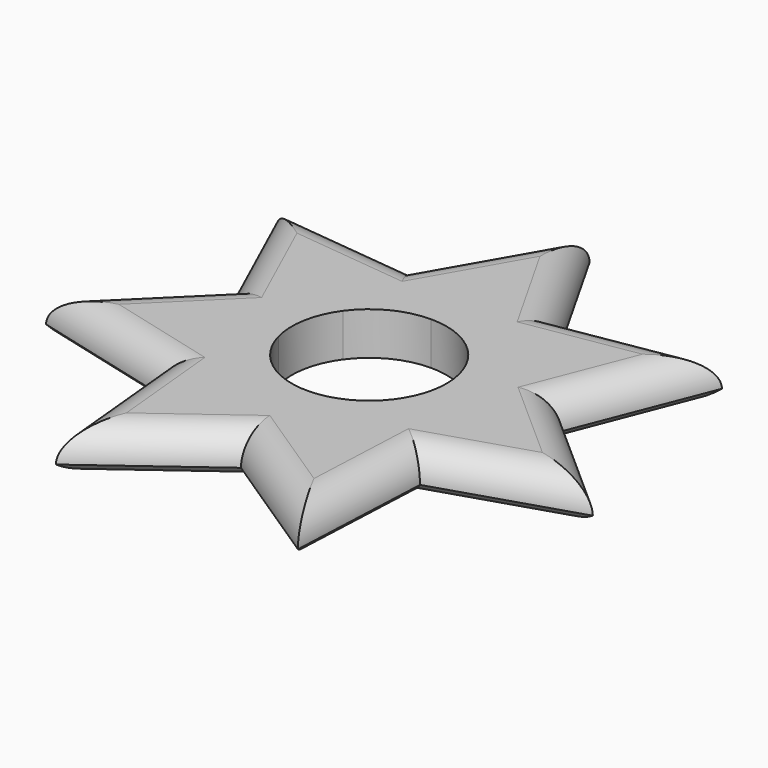
from build123d import *

# Parameters (mm, degrees)
F1_DEPTH      = 7
F2_R          = 5
F3_T4_DEPTH   = 43.6349666374
F3_T9_DEPTH   = 43.6349666374
F3_T14_DEPTH  = 44.4129734555
F3_T19_DEPTH  = 44.4129734555
F3_T24_DEPTH  = 43.6349666396
F3_T29_DEPTH  = 43.6349666396
F3_T34_DEPTH  = 43.6349666396
F3_T39_DEPTH  = 43.6349666396
F3_T44_DEPTH  = 43.6349666396
F3_T49_DEPTH  = 43.6349666396
F3_T54_DEPTH  = 43.6349666396
F3_T59_DEPTH  = 43.6349666418
F3_T64_DEPTH  = 43.6349666418
F3_T69_DEPTH  = 43.6349666396
F3_T75_DEPTH  = 43.6349666374
F3_T79_DEPTH  = 43.6349666374
F3_T86_DEPTH  = 44.4129734555
F3_T90_DEPTH  = 44.4129734555
F3_T97_DEPTH  = 43.6349666396
F3_T101_DEPTH = 43.6349666396
F3_T108_DEPTH = 43.6349666396
F3_T112_DEPTH = 43.6349666396
F3_T119_DEPTH = 43.6349666396
F3_T123_DEPTH = 43.6349666396
F3_T130_DEPTH = 43.6349666396
F3_T134_DEPTH = 43.6349666396
F3_T141_DEPTH = 43.6349666418
F3_T145_DEPTH = 43.6349666418


# Not quite as in the source:
# - a fillet or chamfer that OpenCascade refuses, or shapes differently, is made with other operations: its cross-section is extruded or revolved along the edge and cut away or added


with BuildPart() as f1:
    # F0 (on Top) → F1 (new body)
    with BuildSketch(Plane.XY):
        Polygon((20.4295724883, -40.0952935885), (10.2147862441, -20.0476467942), (0.70880785, -27.0682797275), align=None)
        Polygon((-18.3031489384, -41.1095455939), (-9.1515744692, -20.554772797), (-20.5899370405, -17.5854675412), align=None)
        Polygon((-20.5899370405, -17.5854675412), (-21.7333310915, -5.8234285148), (-43.466662183, -11.6468570296), align=None)
        Polygon((-12.1352549156, 23.8167787844), (0, 22.5), (0, 45), align=None)
        Polygon((-43.466662183, -11.6468570296), (-21.7333310915, -5.8234285148), (-26.62414231, 4.9344931078), align=None)
        Polygon((21.4820715071, -16.4837732251), (10.2147862441, -20.0476467942), (20.4295724883, -40.0952935885), align=None)
        Polygon((-26.62414231, 4.9344931078), (-18.2028823734, 13.2251681766), (-36.4057647469, 26.4503363532), align=None)
        with BuildLine():
            Line((10.2147862441, -20.0476467942), (7.7328428868, -15.176558687))
            ThreePointArc((7.7328428868, -15.176558687), (0.4458732697, -17.0272132106), (-6.927965583, -15.5604654677))
            Line((-6.927965583, -15.5604654677), (-9.1515744692, -20.554772797))
            Line((-9.1515744692, -20.554772797), (10.2147862441, -20.0476467942))
        make_face()
        Polygon((0, 45), (0, 22.5), (11.6571894205, 24.4398058675), align=None)
        Polygon((0.70880785, -27.0682797275), (-9.1515744692, -20.554772797), (-18.3031489384, -41.1095455939), align=None)
        Polygon((-18.2028823734, 13.2251681766), (0, 22.5), (-12.1352549156, 23.8167787844), align=None)
        with BuildLine():
            Line((7.7328428868, -15.176558687), (5.7403470363, -11.2660653986))
            ThreePointArc((5.7403470363, -11.2660653986), (0.3309865905, -12.63986794), (-5.1428597844, -11.5510521989))
            Line((-5.1428597844, -11.5510521989), (-6.927965583, -15.5604654677))
            ThreePointArc((-6.927965583, -15.5604654677), (0.4458732697, -17.0272132106), (7.7328428868, -15.176558687))
        make_face()
        Polygon((34.9715682614, 28.3194176024), (17.4857841307, 14.1597088012), (26.3294034315, 6.3211305052), align=None)
        Polygon((11.6571894205, 24.4398058675), (17.4857841307, 14.1597088012), (34.9715682614, 28.3194176024), align=None)
        Polygon((0, 22.5), (17.4857841307, 14.1597088012), (11.6571894205, 24.4398058675), align=None)
        with BuildLine():
            Line((16.6608370018, -3.5413702277), (12.3678946677, -2.6288771657))
            ThreePointArc((12.3678946677, -2.6288771657), (10.0313189335, -7.6973017427), (5.7403470363, -11.2660653986))
            Line((5.7403470363, -11.2660653986), (7.7328428868, -15.176558687))
            ThreePointArc((7.7328428868, -15.176558687), (13.5132271219, -10.3690638653), (16.6608370018, -3.5413702277))
        make_face()
        Polygon((44.016642033, -9.3560260868), (22.0083210165, -4.6780130434), (21.4820715071, -16.4837732251), align=None)
        Polygon((-20.5899370405, -17.5854675412), (-9.1515744692, -20.554772797), (-21.7333310915, -5.8234285148), align=None)
        Polygon((26.3294034315, 6.3211305052), (22.0083210165, -4.6780130434), (44.016642033, -9.3560260868), align=None)
        with BuildLine():
            ThreePointArc((-12.2133600976, -3.272559975), (-12.4324724808, 2.3042225757), (-10.2293733208, 7.4320747524))
            Line((-10.2293733208, 7.4320747524), (-13.7800269253, 10.0117755983))
            ThreePointArc((-13.7800269253, 10.0117755983), (-16.7478300145, 3.1040268196), (-16.4526629065, -4.4084777391))
            Line((-16.4526629065, -4.4084777391), (-12.2133600976, -3.272559975))
        make_face()
        with BuildLine():
            ThreePointArc((-16.4526629065, -4.4084777391), (-16.7478300145, 3.1040268196), (-13.7800269253, 10.0117755983))
            Line((-13.7800269253, 10.0117755983), (-18.2028823734, 13.2251681766))
            Line((-18.2028823734, 13.2251681766), (-21.7333310915, -5.8234285148))
            Line((-21.7333310915, -5.8234285148), (-16.4526629065, -4.4084777391))
        make_face()
        Polygon((0.70880785, -27.0682797275), (10.2147862441, -20.0476467942), (-9.1515744692, -20.554772797), align=None)
        with BuildLine():
            ThreePointArc((0, 12.6442007918), (5.4434687503, 11.4124695674), (9.82638958, 7.9572533883))
            Line((9.82638958, 7.9572533883), (13.2371660261, 10.7192456959))
            ThreePointArc((13.2371660261, 10.7192456959), (7.3329170413, 15.3737802884), (0, 17.0330500114))
            Line((0, 17.0330500114), (0, 12.6442007918))
        make_face()
        Polygon((-36.4057647469, 26.4503363532), (-18.2028823734, 13.2251681766), (-12.1352549156, 23.8167787844), align=None)
        with BuildLine():
            Line((22.0083210165, -4.6780130434), (16.6608370018, -3.5413702277))
            ThreePointArc((16.6608370018, -3.5413702277), (13.5132271219, -10.3690638653), (7.7328428868, -15.176558687))
            Line((7.7328428868, -15.176558687), (10.2147862441, -20.0476467942))
            Line((10.2147862441, -20.0476467942), (22.0083210165, -4.6780130434))
        make_face()
        with BuildLine():
            ThreePointArc((-10.2293733208, 7.4320747524), (-5.7403470363, 11.2660653986), (0, 12.6442007918))
            Line((0, 12.6442007918), (0, 17.0330500114))
            ThreePointArc((0, 17.0330500114), (-7.7328428868, 15.176558687), (-13.7800269253, 10.0117755983))
            Line((-13.7800269253, 10.0117755983), (-10.2293733208, 7.4320747524))
        make_face()
        with BuildLine():
            ThreePointArc((-13.7800269253, 10.0117755983), (-7.7328428868, 15.176558687), (0, 17.0330500114))
            Line((0, 17.0330500114), (0, 22.5))
            Line((0, 22.5), (-18.2028823734, 13.2251681766))
            Line((-18.2028823734, 13.2251681766), (-13.7800269253, 10.0117755983))
        make_face()
        with BuildLine():
            ThreePointArc((9.82638958, 7.9572533883), (11.9189482877, 4.2207209547), (12.6442007918, 0))
            ThreePointArc((12.6442007918, 0), (12.5749345369, -1.321678878), (12.3678946677, -2.6288771657))
            Line((12.3678946677, -2.6288771657), (16.6608370018, -3.5413702277))
            ThreePointArc((16.6608370018, -3.5413702277), (16.9397411812, -1.7804385425), (17.0330500114, 0))
            ThreePointArc((17.0330500114, 0), (16.0560596602, 5.6857489287), (13.2371660261, 10.7192456959))
            Line((13.2371660261, 10.7192456959), (9.82638958, 7.9572533883))
        make_face()
        with BuildLine():
            Line((-9.1515744692, -20.554772797), (-6.927965583, -15.5604654677))
            ThreePointArc((-6.927965583, -15.5604654677), (-12.952032841, -11.062081087), (-16.4526629065, -4.4084777391))
            Line((-16.4526629065, -4.4084777391), (-21.7333310915, -5.8234285148))
            Line((-21.7333310915, -5.8234285148), (-9.1515744692, -20.554772797))
        make_face()
        Polygon((-21.7333310915, -5.8234285148), (-18.2028823734, 13.2251681766), (-26.62414231, 4.9344931078), align=None)
        with BuildLine():
            Line((-6.927965583, -15.5604654677), (-5.1428597844, -11.5510521989))
            ThreePointArc((-5.1428597844, -11.5510521989), (-9.6147257123, -8.2117515269), (-12.2133600976, -3.272559975))
            Line((-12.2133600976, -3.272559975), (-16.4526629065, -4.4084777391))
            ThreePointArc((-16.4526629065, -4.4084777391), (-12.952032841, -11.062081087), (-6.927965583, -15.5604654677))
        make_face()
        with BuildLine():
            Line((17.4857841307, 14.1597088012), (13.2371660261, 10.7192456959))
            ThreePointArc((13.2371660261, 10.7192456959), (16.0560596602, 5.6857489287), (17.0330500114, 0))
            ThreePointArc((17.0330500114, 0), (16.9397411812, -1.7804385425), (16.6608370018, -3.5413702277))
            Line((16.6608370018, -3.5413702277), (22.0083210165, -4.6780130434))
            Line((22.0083210165, -4.6780130434), (17.4857841307, 14.1597088012))
        make_face()
        Polygon((21.4820715071, -16.4837732251), (22.0083210165, -4.6780130434), (10.2147862441, -20.0476467942), align=None)
        Polygon((26.3294034315, 6.3211305052), (17.4857841307, 14.1597088012), (22.0083210165, -4.6780130434), align=None)
        with BuildLine():
            ThreePointArc((0, 17.0330500114), (7.3329170413, 15.3737802884), (13.2371660261, 10.7192456959))
            Line((13.2371660261, 10.7192456959), (17.4857841307, 14.1597088012))
            Line((17.4857841307, 14.1597088012), (0, 22.5))
            Line((0, 22.5), (0, 17.0330500114))
        make_face()
    extrude(amount=F1_DEPTH)

    # F2
    f2_edges = [f1.edges().sort_by_distance(p)[0] for p in [
        (-24.27051, 25.133558, 7),
        (-6.067627, 34.408389, 7),
        (5.828595, 34.719903, 7),
        (23.314379, 26.379612, 7),
        (35.173023, -1.517448, 7),
        (32.749357, -12.9199, 7),
        (20.955822, -28.289533, 7),
        (10.56919, -33.581787, 7),
        (-8.797171, -34.088913, 7),
        (-19.446543, -29.347507, 7),
        (-32.0283, -14.616162, 7),
        (-35.045402, -3.356182, 7),
        (-31.514954, 15.692415, 7),
        (30.650486, 17.320274, 7),
    ]]
    fillet(f2_edges, radius=F2_R)

    # F3: fillet of radius 5 on 14 edges, made by hand


with BuildPart() as f3_tool2:
    # F3_s3 → F3_t4 (new body)
    with BuildSketch(Plane(origin=(48.4791406288, 8.0671350572, 0), x_dir=(0, 0, 1), z_dir=(-0.9864358685, -0.1641471213, 0))):
        with BuildLine():
            ThreePointArc((0, 18.1948070403), (0.527864045, 20.4308750178), (2, 22.1948070403))
            Line((2, 22.1948070403), (1.94, 22.2748070403))
            ThreePointArc((1.94, 22.2748070403), (1, 22.2948070403), (0, 22.2948070403))
            Line((0, 22.2948070403), (-0.1, 22.1948070403))
            Line((-0.1, 22.1948070403), (-0.1, 18.1948070403))
            Line((-0.1, 18.1948070403), (0, 18.1948070403))
        make_face()
    extrude(amount=F3_T4_DEPTH)

    split(bisect_by=Plane(origin=(19.3073909721, 10.946876879, 0), x_dir=(0, 0, 1), z_dir=(0.8699057819, 0.4932179342, 0)), keep=Keep.TOP)


with BuildPart() as f1_1:
    add(f1.part)

    # F3_t1: cut F3_tool2
    add(f3_tool2.part, mode=Mode.SUBTRACT)


with BuildPart() as f3_tool7:
    # F3_s8 → F3_t9 (new body)
    with BuildSketch(Plane(origin=(-2.7180222094, 4.7938711696, 0), x_dir=(0, 0, 1), z_dir=(-0.4932179342, 0.8699057819, 0))):
        with BuildLine():
            ThreePointArc((0, 18.1948070403), (0.527864045, 20.4308750178), (2, 22.1948070403))
            Line((2, 22.1948070403), (1.94, 22.2748070403))
            ThreePointArc((1.94, 22.2748070403), (1, 22.2948070403), (0, 22.2948070403))
            Line((0, 22.2948070403), (-0.1, 22.1948070403))
            Line((-0.1, 22.1948070403), (-0.1, 18.1948070403))
            Line((-0.1, 18.1948070403), (0, 18.1948070403))
        make_face()
    extrude(amount=F3_T9_DEPTH)

    split(bisect_by=Plane(origin=(-3.6432136829, 21.893753758, 0), x_dir=(0, 0, 1), z_dir=(-0.1641471213, 0.9864358685, 0)), keep=Keep.TOP)


with BuildPart() as f1_2:
    add(f1_1.part)

    # F3_t6: cut F3_tool7
    add(f3_tool7.part, mode=Mode.SUBTRACT)


with BuildPart() as f3_tool12:
    # F3_s13 → F3_t14 (new body)
    with BuildSketch(Plane(origin=(24.3802199512, 42.5579516955, 0), x_dir=(0, 0, 1), z_dir=(-0.4970822148, -0.8677034469, 0))):
        with BuildLine():
            ThreePointArc((0, 18.368699667), (0.527864045, 20.6047676445), (2, 22.368699667))
            Line((2, 22.368699667), (1.94, 22.448699667))
            ThreePointArc((1.94, 22.448699667), (1, 22.468699667), (0, 22.468699667))
            Line((0, 22.468699667), (-0.1, 22.368699667))
            Line((-0.1, 22.368699667), (-0.1, 18.368699667))
            Line((-0.1, 18.368699667), (0, 18.368699667))
        make_face()
    extrude(amount=F3_T14_DEPTH)

    split(bisect_by=Plane(origin=(2.4130308591, 22.2381655463, 0), x_dir=(0, 0, 1), z_dir=(0.10787533, 0.9941644296, 0)), keep=Keep.TOP)


with BuildPart() as f1_3:
    add(f1_2.part)

    # F3_t11: cut F3_tool12
    add(f3_tool12.part, mode=Mode.SUBTRACT)


with BuildPart() as f3_tool17:
    # F3_s18 → F3_t19 (new body)
    with BuildSketch(Plane(origin=(-4.6066414783, 0.4998599377, 0), x_dir=(0, 0, 1), z_dir=(-0.9941644296, 0.10787533, 0))):
        with BuildLine():
            ThreePointArc((0, 18.368699667), (0.527864045, 20.6047676445), (2, 22.368699667))
            Line((2, 22.368699667), (1.94, 22.448699667))
            ThreePointArc((1.94, 22.448699667), (1, 22.468699667), (0, 22.468699667))
            Line((0, 22.468699667), (-0.1, 22.368699667))
            Line((-0.1, 22.368699667), (-0.1, 18.368699667))
            Line((-0.1, 18.368699667), (0, 18.368699667))
        make_face()
    extrude(amount=F3_T19_DEPTH)

    split(bisect_by=Plane(origin=(-19.409397803, 11.1190827731, 0), x_dir=(0, 0, 1), z_dir=(-0.8677034469, 0.4970822148, 0)), keep=Keep.TOP)


with BuildPart() as f1_4:
    add(f1_3.part)

    # F3_t16: cut F3_tool17
    add(f3_tool17.part, mode=Mode.SUBTRACT)


with BuildPart() as f3_tool22:
    # F3_s23 → F3_t24 (new body)
    with BuildSketch(Plane(origin=(-20.3395789734, 44.7393257805, 0), x_dir=(0, 0, 1), z_dir=(0.4138623331, -0.9103394802, 0))):
        with BuildLine():
            ThreePointArc((0, 18.1948070409), (0.527864045, 20.4308750184), (2, 22.1948070409))
            Line((2, 22.1948070409), (1.94, 22.2748070409))
            ThreePointArc((1.94, 22.2748070409), (1, 22.2948070409), (0, 22.2948070409))
            Line((0, 22.2948070409), (-0.1, 22.1948070409))
            Line((-0.1, 22.1948070409), (-0.1, 18.1948070409))
            Line((-0.1, 18.1948070409), (0, 18.1948070409))
        make_face()
    extrude(amount=F3_T24_DEPTH)

    split(bisect_by=Plane(origin=(-15.5709915901, 15.8162473578, 0), x_dir=(0, 0, 1), z_dir=(-0.7015601245, 0.7126102664, 0)), keep=Keep.TOP)


with BuildPart() as f1_5:
    add(f1_4.part)

    # F3_t21: cut F3_tool22
    add(f3_tool22.part, mode=Mode.SUBTRACT)


with BuildPart() as f3_tool27:
    # F3_s28 → F3_t29 (new body)
    with BuildSketch(Plane(origin=(-3.927048056, -3.8661530052, 0), x_dir=(0, 0, 1), z_dir=(-0.7126102664, -0.7015601245, 0))):
        with BuildLine():
            ThreePointArc((0, 18.1948070409), (0.527864045, 20.4308750184), (2, 22.1948070409))
            Line((2, 22.1948070409), (1.94, 22.2748070409))
            ThreePointArc((1.94, 22.2748070409), (1, 22.2948070409), (0, 22.2948070409))
            Line((0, 22.2948070409), (-0.1, 22.1948070409))
            Line((-0.1, 22.1948070409), (-0.1, 18.1948070409))
            Line((-0.1, 18.1948070409), (0, 18.1948070409))
        make_face()
    extrude(amount=F3_T29_DEPTH)

    split(bisect_by=Plane(origin=(-20.2048091048, -9.1855946253, 0), x_dir=(0, 0, 1), z_dir=(-0.9103394802, -0.4138623331, 0)), keep=Keep.TOP)


with BuildPart() as f1_6:
    add(f1_5.part)

    # F3_t26: cut F3_tool27
    add(f3_tool27.part, mode=Mode.SUBTRACT)


with BuildPart() as f3_tool32:
    # F3_s33 → F3_t34 (new body)
    with BuildSketch(Plane(origin=(-47.5690981419, 12.3485483386, 0), x_dir=(0, 0, 1), z_dir=(0.9679186559, -0.2512637569, 0))):
        with BuildLine():
            ThreePointArc((0, 18.1948070409), (0.527864045, 20.4308750184), (2, 22.1948070409))
            Line((2, 22.1948070409), (1.94, 22.2748070409))
            ThreePointArc((1.94, 22.2748070409), (1, 22.2948070409), (0, 22.2948070409))
            Line((0, 22.2948070409), (-0.1, 22.1948070409))
            Line((-0.1, 22.1948070409), (-0.1, 18.1948070409))
            Line((-0.1, 18.1948070409), (0, 18.1948070409))
        make_face()
    extrude(amount=F3_T34_DEPTH)

    split(bisect_by=Plane(origin=(-22.090675276, -2.147446258, 0), x_dir=(0, 0, 1), z_dir=(-0.9953082825, -0.0967544459, 0)), keep=Keep.TOP)


with BuildPart() as f1_7:
    add(f1_6.part)

    # F3_t31: cut F3_tool32
    add(f3_tool32.part, mode=Mode.SUBTRACT)


with BuildPart() as f3_tool37:
    # F3_s38 → F3_t39 (new body)
    with BuildSketch(Plane(origin=(0.5331937761, -5.4849384583, 0), x_dir=(0, 0, 1), z_dir=(0.0967544459, -0.9953082825, 0))):
        with BuildLine():
            ThreePointArc((0, 18.1948070409), (0.527864045, 20.4308750184), (2, 22.1948070409))
            Line((2, 22.1948070409), (1.94, 22.2748070409))
            ThreePointArc((1.94, 22.2748070409), (1, 22.2948070409), (0, 22.2948070409))
            Line((0, 22.2948070409), (-0.1, 22.1948070409))
            Line((-0.1, 22.1948070409), (-0.1, 18.1948070409))
            Line((-0.1, 18.1948070409), (0, 18.1948070409))
        make_face()
    extrude(amount=F3_T39_DEPTH)

    split(bisect_by=Plane(origin=(-5.5767506003, -21.4827677994, 0), x_dir=(0, 0, 1), z_dir=(-0.2512637569, -0.9679186559, 0)), keep=Keep.TOP)


with BuildPart() as f1_8:
    add(f1_7.part)

    # F3_t36: cut F3_tool37
    add(f3_tool37.part, mode=Mode.SUBTRACT)


with BuildPart() as f3_tool42:
    # F3_s43 → F3_t44 (new body)
    with BuildSketch(Plane(origin=(-39.5328279158, -29.1969392418, 0), x_dir=(0, 0, 1), z_dir=(0.804399561, 0.5940886687, 0))):
        with BuildLine():
            ThreePointArc((2, 22.1948070409), (0.527864045, 20.4308750184), (0, 18.1948070409))
            Line((0, 18.1948070409), (-0.1, 18.1948070409))
            Line((-0.1, 18.1948070409), (-0.1, 22.1948070409))
            Line((-0.1, 22.1948070409), (0, 22.2948070409))
            ThreePointArc((0, 22.2948070409), (1, 22.2948070409), (1.94, 22.2748070409))
            Line((1.94, 22.2748070409), (2, 22.1948070409))
        make_face()
    extrude(amount=F3_T44_DEPTH)

    split(bisect_by=Plane(origin=(-12.2332332164, -18.5191107955, 0), x_dir=(0, 0, 1), z_dir=(-0.5511754706, -0.8343893579, 0)), keep=Keep.TOP)


with BuildPart() as f1_9:
    add(f1_8.part)

    # F3_t41: cut F3_tool42
    add(f3_tool42.part, mode=Mode.SUBTRACT)


with BuildPart() as f3_tool47:
    # F3_s48 → F3_t49 (new body)
    with BuildSketch(Plane(origin=(4.5981474874, -3.0374142256, 0), x_dir=(0, 0, 1), z_dir=(0.8343893579, -0.5511754706, 0))):
        with BuildLine():
            ThreePointArc((2, 22.1948070409), (0.527864045, 20.4308750184), (0, 18.1948070409))
            Line((0, 18.1948070409), (-0.1, 18.1948070409))
            Line((-0.1, 18.1948070409), (-0.1, 22.1948070409))
            Line((-0.1, 22.1948070409), (0, 22.2948070409))
            ThreePointArc((0, 22.2948070409), (1, 22.2948070409), (1.94, 22.2748070409))
            Line((1.94, 22.2748070409), (2, 22.1948070409))
        make_face()
    extrude(amount=F3_T49_DEPTH)

    split(bisect_by=Plane(origin=(13.1856833677, -17.8534930394, 0), x_dir=(0, 0, 1), z_dir=(0.5940886687, -0.804399561, 0)), keep=Keep.TOP)


with BuildPart() as f1_10:
    add(f1_9.part)

    # F3_t46: cut F3_tool47
    add(f3_tool47.part, mode=Mode.SUBTRACT)


with BuildPart() as f3_tool52:
    # F3_s53 → F3_t54 (new body)
    with BuildSketch(Plane(origin=(5.2542221736, 1.6619250417, 0), x_dir=(0, 0, 1), z_dir=(0.9534420281, 0.3015763571, 0))):
        with BuildLine():
            ThreePointArc((0, 18.1948070409), (0.527864045, 20.4308750184), (2, 22.1948070409))
            Line((2, 22.1948070409), (1.94, 22.2748070409))
            ThreePointArc((1.94, 22.2748070409), (1, 22.2948070409), (0, 22.2948070409))
            Line((0, 22.2948070409), (-0.1, 22.1948070409))
            Line((-0.1, 22.1948070409), (-0.1, 18.1948070409))
            Line((-0.1, 18.1948070409), (0, 18.1948070409))
        make_face()
    extrude(amount=F3_T54_DEPTH)

    split(bisect_by=Plane(origin=(22.1727894267, -0.9883666429, 0), x_dir=(0, 0, 1), z_dir=(0.9990079835, -0.0445314366, 0)), keep=Keep.TOP)


with BuildPart() as f1_11:
    add(f1_10.part)

    # F3_t51: cut F3_tool52
    add(f3_tool52.part, mode=Mode.SUBTRACT)


with BuildPart() as f3_tool57:
    # F3_s58 → F3_t59 (new body)
    with BuildSketch(Plane(origin=(36.7782531622, -32.5985557719, 0), x_dir=(0, 0, 1), z_dir=(-0.7483504787, 0.663303521, 0))):
        with BuildLine():
            ThreePointArc((0, 18.1948070415), (0.527864045, 20.430875019), (2, 22.1948070415))
            Line((2, 22.1948070415), (1.94, 22.2748070415))
            ThreePointArc((1.94, 22.2748070415), (1, 22.2948070415), (0, 22.2948070415))
            Line((0, 22.2948070415), (-0.1, 22.1948070415))
            Line((-0.1, 22.1948070415), (-0.1, 18.1948070415))
            Line((-0.1, 18.1948070415), (0, 18.1948070415))
        make_face()
    extrude(amount=F3_T59_DEPTH)

    split(bisect_by=Plane(origin=(20.6578559964, -8.1155680787, 0), x_dir=(0, 0, 1), z_dir=(0.9307517726, -0.3656516618, 0)), keep=Keep.TOP)


with BuildPart() as f1_12:
    add(f1_11.part)

    # F3_t56: cut F3_tool57
    add(f3_tool57.part, mode=Mode.SUBTRACT)


with BuildPart() as f3_tool62:
    # F3_s63 → F3_t64 (new body)
    with BuildSketch(Plane(origin=(2.0150308168, 5.1291808579, 0), x_dir=(0, 0, 1), z_dir=(0.3656516618, 0.9307517726, 0))):
        with BuildLine():
            ThreePointArc((0, 18.1948070415), (0.527864045, 20.430875019), (2, 22.1948070415))
            Line((2, 22.1948070415), (1.94, 22.2748070415))
            ThreePointArc((1.94, 22.2748070415), (1, 22.2948070415), (0, 22.2948070415))
            Line((0, 22.2948070415), (-0.1, 22.1948070415))
            Line((-0.1, 22.1948070415), (-0.1, 18.1948070415))
            Line((-0.1, 18.1948070415), (0, 18.1948070415))
        make_face()
    extrude(amount=F3_T64_DEPTH)

    split(bisect_by=Plane(origin=(14.7218936583, 16.6094944752, 0), x_dir=(0, 0, 1), z_dir=(0.663303521, 0.7483504787, 0)), keep=Keep.TOP)


with BuildPart() as f1_13:
    add(f1_12.part)

    # F3_t61: cut F3_tool62
    add(f3_tool62.part, mode=Mode.SUBTRACT)


with BuildPart() as f3_tool67:
    # F3_s68 → F3_t69 (new body)
    with BuildSketch(Plane(origin=(-2.1885313046, -49.0970067808, 0), x_dir=(0, 0, 1), z_dir=(0.0445314366, 0.9990079835, 0))):
        with BuildLine():
            ThreePointArc((0, 18.1948070409), (0.527864045, 20.4308750184), (2, 22.1948070409))
            Line((2, 22.1948070409), (1.94, 22.2748070409))
            ThreePointArc((1.94, 22.2748070409), (1, 22.2948070409), (0, 22.2948070409))
            Line((0, 22.2948070409), (-0.1, 22.1948070409))
            Line((-0.1, 22.1948070409), (-0.1, 18.1948070409))
            Line((-0.1, 18.1948070409), (0, 18.1948070409))
        make_face()
    extrude(amount=F3_T69_DEPTH)

    split(bisect_by=Plane(origin=(6.6934290529, -21.1614618374, 0), x_dir=(0, 0, 1), z_dir=(0.3015763571, -0.9534420281, 0)), keep=Keep.TOP)


with BuildPart() as f1_14:
    add(f1_13.part)

    # F3_t66: cut F3_tool67
    add(f3_tool67.part, mode=Mode.SUBTRACT)


with BuildPart() as f3_tool73:
    # F3_s74 → F3_t75 (new body)
    with BuildSketch(Plane(origin=(48.4791406288, 8.0671350572, 0), x_dir=(0, 0, 1), z_dir=(-0.9864358685, -0.1641471213, 0))):
        with BuildLine():
            ThreePointArc((0, 18.1948070403), (0.527864045, 20.4308750178), (2, 22.1948070403))
            Line((2, 22.1948070403), (1.94, 22.2748070403))
            ThreePointArc((1.94, 22.2748070403), (1, 22.2948070403), (0, 22.2948070403))
            Line((0, 22.2948070403), (-0.1, 22.1948070403))
            Line((-0.1, 22.1948070403), (-0.1, 18.1948070403))
            Line((-0.1, 18.1948070403), (0, 18.1948070403))
        make_face()
    extrude(amount=F3_T75_DEPTH)

    split(bisect_by=Plane(origin=(19.3073909721, 10.946876879, 0), x_dir=(0, 0, 1), z_dir=(-0.8699057819, -0.4932179342, 0)), keep=Keep.TOP)


with BuildPart() as f3_tool77:
    # F3_s78 → F3_t79 (new body)
    with BuildSketch(Plane(origin=(-2.7180222094, 4.7938711696, 0), x_dir=(0, 0, 1), z_dir=(-0.4932179342, 0.8699057819, 0))):
        with BuildLine():
            ThreePointArc((0, 18.1948070403), (0.527864045, 20.4308750178), (2, 22.1948070403))
            Line((2, 22.1948070403), (1.94, 22.2748070403))
            ThreePointArc((1.94, 22.2748070403), (1, 22.2948070403), (0, 22.2948070403))
            Line((0, 22.2948070403), (-0.1, 22.1948070403))
            Line((-0.1, 22.1948070403), (-0.1, 18.1948070403))
            Line((-0.1, 18.1948070403), (0, 18.1948070403))
        make_face()
    extrude(amount=F3_T79_DEPTH)

    split(bisect_by=Plane(origin=(-3.6432136829, 21.893753758, 0), x_dir=(0, 0, 1), z_dir=(0.1641471213, -0.9864358685, 0)), keep=Keep.TOP)


with BuildPart() as f3_tool73_1:
    add(f3_tool73.part)

    # F3_t81: intersect F3_tool77
    add(f3_tool77.part, mode=Mode.INTERSECT)


with BuildPart() as f1_15:
    add(f1_14.part)

    # F3_t71: cut F3_tool73
    add(f3_tool73_1.part, mode=Mode.SUBTRACT)


with BuildPart() as f3_tool84:
    # F3_s85 → F3_t86 (new body)
    with BuildSketch(Plane(origin=(24.3802199512, 42.5579516955, 0), x_dir=(0, 0, 1), z_dir=(-0.4970822148, -0.8677034469, 0))):
        with BuildLine():
            ThreePointArc((0, 18.368699667), (0.527864045, 20.6047676445), (2, 22.368699667))
            Line((2, 22.368699667), (1.94, 22.448699667))
            ThreePointArc((1.94, 22.448699667), (1, 22.468699667), (0, 22.468699667))
            Line((0, 22.468699667), (-0.1, 22.368699667))
            Line((-0.1, 22.368699667), (-0.1, 18.368699667))
            Line((-0.1, 18.368699667), (0, 18.368699667))
        make_face()
    extrude(amount=F3_T86_DEPTH)

    split(bisect_by=Plane(origin=(2.4130308591, 22.2381655463, 0), x_dir=(0, 0, 1), z_dir=(-0.10787533, -0.9941644296, 0)), keep=Keep.TOP)


with BuildPart() as f3_tool88:
    # F3_s89 → F3_t90 (new body)
    with BuildSketch(Plane(origin=(-4.6066414783, 0.4998599377, 0), x_dir=(0, 0, 1), z_dir=(-0.9941644296, 0.10787533, 0))):
        with BuildLine():
            ThreePointArc((0, 18.368699667), (0.527864045, 20.6047676445), (2, 22.368699667))
            Line((2, 22.368699667), (1.94, 22.448699667))
            ThreePointArc((1.94, 22.448699667), (1, 22.468699667), (0, 22.468699667))
            Line((0, 22.468699667), (-0.1, 22.368699667))
            Line((-0.1, 22.368699667), (-0.1, 18.368699667))
            Line((-0.1, 18.368699667), (0, 18.368699667))
        make_face()
    extrude(amount=F3_T90_DEPTH)

    split(bisect_by=Plane(origin=(-19.409397803, 11.1190827731, 0), x_dir=(0, 0, 1), z_dir=(0.8677034469, -0.4970822148, 0)), keep=Keep.TOP)


with BuildPart() as f3_tool84_1:
    add(f3_tool84.part)

    # F3_t92: intersect F3_tool88
    add(f3_tool88.part, mode=Mode.INTERSECT)


with BuildPart() as f1_16:
    add(f1_15.part)

    # F3_t82: cut F3_tool84
    add(f3_tool84_1.part, mode=Mode.SUBTRACT)


with BuildPart() as f3_tool95:
    # F3_s96 → F3_t97 (new body)
    with BuildSketch(Plane(origin=(-20.3395789734, 44.7393257805, 0), x_dir=(0, 0, 1), z_dir=(0.4138623331, -0.9103394802, 0))):
        with BuildLine():
            ThreePointArc((0, 18.1948070409), (0.527864045, 20.4308750184), (2, 22.1948070409))
            Line((2, 22.1948070409), (1.94, 22.2748070409))
            ThreePointArc((1.94, 22.2748070409), (1, 22.2948070409), (0, 22.2948070409))
            Line((0, 22.2948070409), (-0.1, 22.1948070409))
            Line((-0.1, 22.1948070409), (-0.1, 18.1948070409))
            Line((-0.1, 18.1948070409), (0, 18.1948070409))
        make_face()
    extrude(amount=F3_T97_DEPTH)

    split(bisect_by=Plane(origin=(-15.5709915901, 15.8162473578, 0), x_dir=(0, 0, 1), z_dir=(0.7015601245, -0.7126102664, 0)), keep=Keep.TOP)


with BuildPart() as f3_tool99:
    # F3_s100 → F3_t101 (new body)
    with BuildSketch(Plane(origin=(-3.927048056, -3.8661530052, 0), x_dir=(0, 0, 1), z_dir=(-0.7126102664, -0.7015601245, 0))):
        with BuildLine():
            ThreePointArc((0, 18.1948070409), (0.527864045, 20.4308750184), (2, 22.1948070409))
            Line((2, 22.1948070409), (1.94, 22.2748070409))
            ThreePointArc((1.94, 22.2748070409), (1, 22.2948070409), (0, 22.2948070409))
            Line((0, 22.2948070409), (-0.1, 22.1948070409))
            Line((-0.1, 22.1948070409), (-0.1, 18.1948070409))
            Line((-0.1, 18.1948070409), (0, 18.1948070409))
        make_face()
    extrude(amount=F3_T101_DEPTH)

    split(bisect_by=Plane(origin=(-20.2048091048, -9.1855946253, 0), x_dir=(0, 0, 1), z_dir=(0.9103394802, 0.4138623331, 0)), keep=Keep.TOP)


with BuildPart() as f3_tool95_1:
    add(f3_tool95.part)

    # F3_t103: intersect F3_tool99
    add(f3_tool99.part, mode=Mode.INTERSECT)


with BuildPart() as f1_17:
    add(f1_16.part)

    # F3_t93: cut F3_tool95
    add(f3_tool95_1.part, mode=Mode.SUBTRACT)


with BuildPart() as f3_tool106:
    # F3_s107 → F3_t108 (new body)
    with BuildSketch(Plane(origin=(-47.5690981419, 12.3485483386, 0), x_dir=(0, 0, 1), z_dir=(0.9679186559, -0.2512637569, 0))):
        with BuildLine():
            ThreePointArc((0, 18.1948070409), (0.527864045, 20.4308750184), (2, 22.1948070409))
            Line((2, 22.1948070409), (1.94, 22.2748070409))
            ThreePointArc((1.94, 22.2748070409), (1, 22.2948070409), (0, 22.2948070409))
            Line((0, 22.2948070409), (-0.1, 22.1948070409))
            Line((-0.1, 22.1948070409), (-0.1, 18.1948070409))
            Line((-0.1, 18.1948070409), (0, 18.1948070409))
        make_face()
    extrude(amount=F3_T108_DEPTH)

    split(bisect_by=Plane(origin=(-22.090675276, -2.147446258, 0), x_dir=(0, 0, 1), z_dir=(0.9953082825, 0.0967544459, 0)), keep=Keep.TOP)


with BuildPart() as f3_tool110:
    # F3_s111 → F3_t112 (new body)
    with BuildSketch(Plane(origin=(0.5331937761, -5.4849384583, 0), x_dir=(0, 0, 1), z_dir=(0.0967544459, -0.9953082825, 0))):
        with BuildLine():
            ThreePointArc((0, 18.1948070409), (0.527864045, 20.4308750184), (2, 22.1948070409))
            Line((2, 22.1948070409), (1.94, 22.2748070409))
            ThreePointArc((1.94, 22.2748070409), (1, 22.2948070409), (0, 22.2948070409))
            Line((0, 22.2948070409), (-0.1, 22.1948070409))
            Line((-0.1, 22.1948070409), (-0.1, 18.1948070409))
            Line((-0.1, 18.1948070409), (0, 18.1948070409))
        make_face()
    extrude(amount=F3_T112_DEPTH)

    split(bisect_by=Plane(origin=(-5.5767506003, -21.4827677994, 0), x_dir=(0, 0, 1), z_dir=(0.2512637569, 0.9679186559, 0)), keep=Keep.TOP)


with BuildPart() as f3_tool106_1:
    add(f3_tool106.part)

    # F3_t114: intersect F3_tool110
    add(f3_tool110.part, mode=Mode.INTERSECT)


with BuildPart() as f1_18:
    add(f1_17.part)

    # F3_t104: cut F3_tool106
    add(f3_tool106_1.part, mode=Mode.SUBTRACT)


with BuildPart() as f3_tool117:
    # F3_s118 → F3_t119 (new body)
    with BuildSketch(Plane(origin=(4.5981474874, -3.0374142256, 0), x_dir=(0, 0, 1), z_dir=(0.8343893579, -0.5511754706, 0))):
        with BuildLine():
            ThreePointArc((2, 22.1948070409), (0.527864045, 20.4308750184), (0, 18.1948070409))
            Line((0, 18.1948070409), (-0.1, 18.1948070409))
            Line((-0.1, 18.1948070409), (-0.1, 22.1948070409))
            Line((-0.1, 22.1948070409), (0, 22.2948070409))
            ThreePointArc((0, 22.2948070409), (1, 22.2948070409), (1.94, 22.2748070409))
            Line((1.94, 22.2748070409), (2, 22.1948070409))
        make_face()
    extrude(amount=F3_T119_DEPTH)

    split(bisect_by=Plane(origin=(13.1856833677, -17.8534930394, 0), x_dir=(0, 0, 1), z_dir=(-0.5940886687, 0.804399561, 0)), keep=Keep.TOP)


with BuildPart() as f3_tool121:
    # F3_s122 → F3_t123 (new body)
    with BuildSketch(Plane(origin=(-39.5328279158, -29.1969392418, 0), x_dir=(0, 0, 1), z_dir=(0.804399561, 0.5940886687, 0))):
        with BuildLine():
            ThreePointArc((2, 22.1948070409), (0.527864045, 20.4308750184), (0, 18.1948070409))
            Line((0, 18.1948070409), (-0.1, 18.1948070409))
            Line((-0.1, 18.1948070409), (-0.1, 22.1948070409))
            Line((-0.1, 22.1948070409), (0, 22.2948070409))
            ThreePointArc((0, 22.2948070409), (1, 22.2948070409), (1.94, 22.2748070409))
            Line((1.94, 22.2748070409), (2, 22.1948070409))
        make_face()
    extrude(amount=F3_T123_DEPTH)

    split(bisect_by=Plane(origin=(-12.2332332164, -18.5191107955, 0), x_dir=(0, 0, 1), z_dir=(0.5511754706, 0.8343893579, 0)), keep=Keep.TOP)


with BuildPart() as f3_tool117_1:
    add(f3_tool117.part)

    # F3_t125: intersect F3_tool121
    add(f3_tool121.part, mode=Mode.INTERSECT)


with BuildPart() as f1_19:
    add(f1_18.part)

    # F3_t115: cut F3_tool117
    add(f3_tool117_1.part, mode=Mode.SUBTRACT)


with BuildPart() as f3_tool128:
    # F3_s129 → F3_t130 (new body)
    with BuildSketch(Plane(origin=(-2.1885313046, -49.0970067808, 0), x_dir=(0, 0, 1), z_dir=(0.0445314366, 0.9990079835, 0))):
        with BuildLine():
            ThreePointArc((0, 18.1948070409), (0.527864045, 20.4308750184), (2, 22.1948070409))
            Line((2, 22.1948070409), (1.94, 22.2748070409))
            ThreePointArc((1.94, 22.2748070409), (1, 22.2948070409), (0, 22.2948070409))
            Line((0, 22.2948070409), (-0.1, 22.1948070409))
            Line((-0.1, 22.1948070409), (-0.1, 18.1948070409))
            Line((-0.1, 18.1948070409), (0, 18.1948070409))
        make_face()
    extrude(amount=F3_T130_DEPTH)

    split(bisect_by=Plane(origin=(6.6934290529, -21.1614618374, 0), x_dir=(0, 0, 1), z_dir=(-0.3015763571, 0.9534420281, 0)), keep=Keep.TOP)


with BuildPart() as f3_tool132:
    # F3_s133 → F3_t134 (new body)
    with BuildSketch(Plane(origin=(5.2542221736, 1.6619250417, 0), x_dir=(0, 0, 1), z_dir=(0.9534420281, 0.3015763571, 0))):
        with BuildLine():
            ThreePointArc((0, 18.1948070409), (0.527864045, 20.4308750184), (2, 22.1948070409))
            Line((2, 22.1948070409), (1.94, 22.2748070409))
            ThreePointArc((1.94, 22.2748070409), (1, 22.2948070409), (0, 22.2948070409))
            Line((0, 22.2948070409), (-0.1, 22.1948070409))
            Line((-0.1, 22.1948070409), (-0.1, 18.1948070409))
            Line((-0.1, 18.1948070409), (0, 18.1948070409))
        make_face()
    extrude(amount=F3_T134_DEPTH)

    split(bisect_by=Plane(origin=(22.1727894267, -0.9883666429, 0), x_dir=(0, 0, 1), z_dir=(-0.9990079835, 0.0445314366, 0)), keep=Keep.TOP)


with BuildPart() as f3_tool128_1:
    add(f3_tool128.part)

    # F3_t136: intersect F3_tool132
    add(f3_tool132.part, mode=Mode.INTERSECT)


with BuildPart() as f1_20:
    add(f1_19.part)

    # F3_t126: cut F3_tool128
    add(f3_tool128_1.part, mode=Mode.SUBTRACT)


with BuildPart() as f3_tool139:
    # F3_s140 → F3_t141 (new body)
    with BuildSketch(Plane(origin=(36.7782531622, -32.5985557719, 0), x_dir=(0, 0, 1), z_dir=(-0.7483504787, 0.663303521, 0))):
        with BuildLine():
            ThreePointArc((0, 18.1948070415), (0.527864045, 20.430875019), (2, 22.1948070415))
            Line((2, 22.1948070415), (1.94, 22.2748070415))
            ThreePointArc((1.94, 22.2748070415), (1, 22.2948070415), (0, 22.2948070415))
            Line((0, 22.2948070415), (-0.1, 22.1948070415))
            Line((-0.1, 22.1948070415), (-0.1, 18.1948070415))
            Line((-0.1, 18.1948070415), (0, 18.1948070415))
        make_face()
    extrude(amount=F3_T141_DEPTH)

    split(bisect_by=Plane(origin=(20.6578559964, -8.1155680787, 0), x_dir=(0, 0, 1), z_dir=(-0.9307517726, 0.3656516618, 0)), keep=Keep.TOP)


with BuildPart() as f3_tool143:
    # F3_s144 → F3_t145 (new body)
    with BuildSketch(Plane(origin=(2.0150308168, 5.1291808579, 0), x_dir=(0, 0, 1), z_dir=(0.3656516618, 0.9307517726, 0))):
        with BuildLine():
            ThreePointArc((0, 18.1948070415), (0.527864045, 20.430875019), (2, 22.1948070415))
            Line((2, 22.1948070415), (1.94, 22.2748070415))
            ThreePointArc((1.94, 22.2748070415), (1, 22.2948070415), (0, 22.2948070415))
            Line((0, 22.2948070415), (-0.1, 22.1948070415))
            Line((-0.1, 22.1948070415), (-0.1, 18.1948070415))
            Line((-0.1, 18.1948070415), (0, 18.1948070415))
        make_face()
    extrude(amount=F3_T145_DEPTH)

    split(bisect_by=Plane(origin=(14.7218936583, 16.6094944752, 0), x_dir=(0, 0, 1), z_dir=(-0.663303521, -0.7483504787, 0)), keep=Keep.TOP)


with BuildPart() as f3_tool139_1:
    add(f3_tool139.part)

    # F3_t147: intersect F3_tool143
    add(f3_tool143.part, mode=Mode.INTERSECT)


with BuildPart() as f1_21:
    add(f1_20.part)

    # F3_t137: cut F3_tool139
    add(f3_tool139_1.part, mode=Mode.SUBTRACT)


solid = f1_21.part
